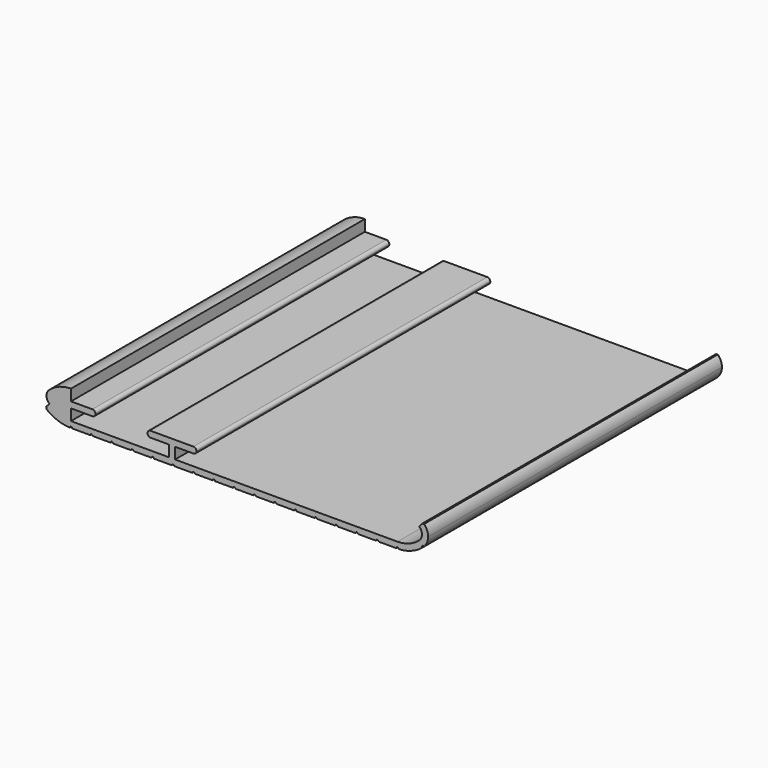
from build123d import *

# Parameters (mm, degrees)
F1_DEPTH  = 90
F2_T      = -1.5
F4_DEPTH  = 90.001
F6_DEPTH  = 90
F8_DEPTH  = 90
F9_R      = 0.74999
F10_R     = 0.3
F11_DEPTH = 90.001


# Not quite as in the source:
# - a fillet or chamfer is up to 0.001 mm smaller than in the source, because OpenCascade refuses the exact size


with BuildPart() as f1:
    # F0 (on Front) → F1 (new body)
    with BuildSketch(Plane.XZ):
        with BuildLine():
            Line((40, 5), (0, 5))
            Line((0, 5), (-40, 5))
            ThreePointArc((-40, 5), (-43.3649329819, 4.389821285), (-46.301369863, 2.6369863014))
            ThreePointArc((-46.301369863, 2.6369863014), (-47.1862826711, 1.4483103051), (-47.5, 0))
            ThreePointArc((-47.5, 0), (-47.1862826711, -1.4483103051), (-46.301369863, -2.6369863014))
            ThreePointArc((-46.301369863, -2.6369863014), (-43.3649329819, -4.389821285), (-40, -5))
            Line((-40, -5), (0, -5))
            Line((0, -5), (40, -5))
            ThreePointArc((40, -5), (43.3649329819, -4.389821285), (46.301369863, -2.6369863014))
            ThreePointArc((46.301369863, -2.6369863014), (47.1862826711, -1.4483103051), (47.5, 0))
            ThreePointArc((47.5, 0), (47.1862826711, 1.4483103051), (46.301369863, 2.6369863014))
            ThreePointArc((46.301369863, 2.6369863014), (43.3649329819, 4.389821285), (40, 5))
        make_face()
    extrude(amount=F1_DEPTH)

    # F2
    f2_openings = [f1.faces().sort_by_distance(p)[0] for p in [
        (0, -90, 0),
        (0, 0, 0),
    ]]
    offset(amount=F2_T, openings=f2_openings)

    # F3 (on Front) → F4 (cut, through all)
    with BuildSketch(Plane.XZ):
        Polygon((-44, 0), (44, 0), (52.7272727273, 10), (-47.5, 10), (-47.5, -4.0104166667), align=None)
    extrude(amount=F4_DEPTH, mode=Mode.SUBTRACT)

    # F5 (on Front) → F6 (join, through all)
    with BuildSketch(Plane.XZ):
        with BuildLine():
            ThreePointArc((-40, 3.5), (-42.8382478195, 2.9853275187), (-45.3150684932, 1.5068493151))
            ThreePointArc((-45.3150684932, 1.5068493151), (-46, 0), (-45.3150684932, -1.5068493151))
            ThreePointArc((-45.3150684932, -1.5068493151), (-42.8382478195, -2.9853275187), (-40, -3.5))
            Line((-40, -3.5), (-40, -0.75))
            Line((-40, -0.75), (-34, -0.75))
            Line((-34, -0.75), (-34, 0.75))
            Line((-34, 0.75), (-40, 0.75))
            Line((-40, 0.75), (-40, 3.5))
        make_face()
    extrude(amount=F6_DEPTH)

    # F7 (on Front) → F8 (join, through all)
    with BuildSketch(Plane.XZ):
        Polygon((-16, -0.75), (-16, -3.5), (-14.5, -3.5), (-14.5, -0.75), (-9.25, -0.75), (-9.25, 0.75), (-21.25, 0.75), (-21.25, -0.75), align=None)
    extrude(amount=F8_DEPTH)

    # F9 (radius 0.75 in the source; OpenCascade refuses exactly that, so slightly less here)
    f9_edges = [f1.edges().sort_by_distance(p)[0] for p in [
        (-34, -45, 0.75),
        (-34, -45, -0.75),
        (-9.25, -45, 0.75),
        (-9.25, -45, -0.75),
        (-21.25, -45, 0.75),
        (-21.25, -45, -0.75),
    ]]
    fillet(f9_edges, radius=F9_R)

    # F10 (on Front) → F11 (cut, through all)
    with BuildSketch(Plane.XZ):
        with Locations((40, -5)):
            Circle(F10_R)
        with Locations((35, -5)):
            Circle(F10_R)
        with Locations((30, -5)):
            Circle(F10_R)
        with Locations((25, -5)):
            Circle(F10_R)
        with Locations((20, -5)):
            Circle(F10_R)
        with Locations((15, -5)):
            Circle(F10_R)
        with Locations((10, -5)):
            Circle(F10_R)
        with Locations((5, -5)):
            Circle(F10_R)
        with Locations((0, -5)):
            Circle(F10_R)
        with Locations((46.301369863, -2.6369863014)):
            Circle(F10_R)
        with Locations((-5, -5)):
            Circle(F10_R)
        with Locations((-10, -5)):
            Circle(F10_R)
        with Locations((-15, -5)):
            Circle(F10_R)
        with Locations((-20, -5)):
            Circle(F10_R)
        with Locations((-25, -5)):
            Circle(F10_R)
        with Locations((-30, -5)):
            Circle(F10_R)
        with Locations((-35, -5)):
            Circle(F10_R)
        with Locations((-40, -5)):
            Circle(F10_R)
        with Locations((46.301369863, 2.6369863014)):
            Circle(F10_R)
        with Locations((-46.301369863, -2.6369863014)):
            Circle(F10_R)
    extrude(amount=F11_DEPTH, mode=Mode.SUBTRACT)


solid = f1.part
